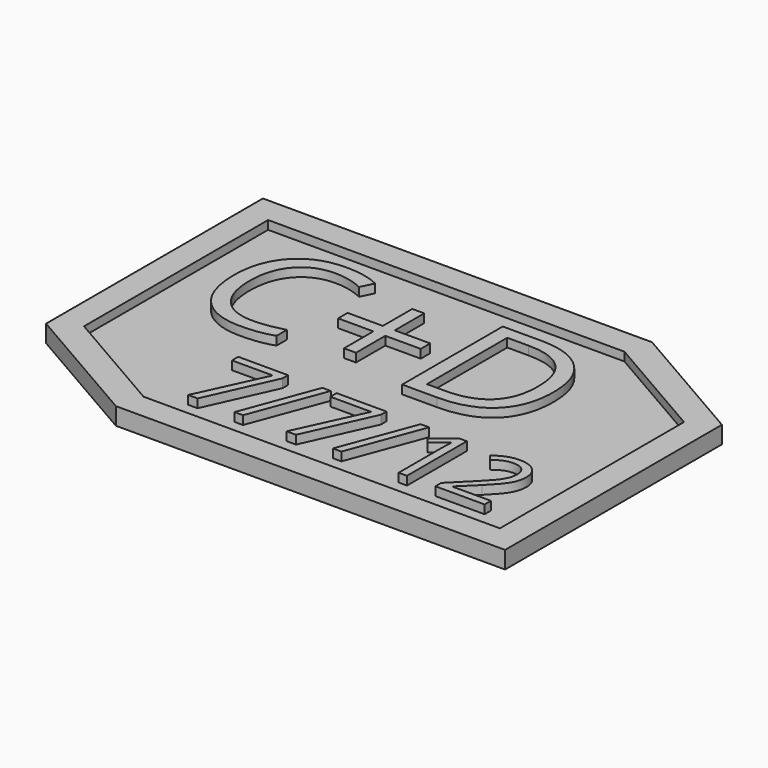
from build123d import *

# Parameters (mm, degrees)
F0_W           = 60
F0_H           = 40
F1_DEPTH       = 1
F2_SIZE2       = 8.6602540378
F2_SIZE        = 15
F2_2_SIZE2     = 8.6602540378
F2_2_SIZE      = 15
F4_DEPTH       = 1
F5_TEXT_SIZE   = 20.360840588
F5_TEXT_SIZE_2 = 12.11661535
F6_DEPTH       = 1


# Not quite as in the source:
# - Text() gives the source's letters only with a copy of the font that has no kerning and outlines rounded to 1/6400 em; it was checked with that copy


with BuildPart() as f1:
    # F0 (on Top) → F1 (new body)
    with BuildSketch(Plane.XY):
        with Locations((30, 20)):
            Rectangle(F0_W, F0_H)
    extrude(amount=F1_DEPTH)

    # F2
    f2_edges = [f1.edges().sort_by_distance(p)[0] for p in [
        (0, 0, 0.5),
    ]]
    f2_side = f1.faces().sort_by_distance((30, 0, 0.5))[0]
    chamfer(f2_edges, length=F2_SIZE, length2=F2_SIZE2, reference=f2_side)

    # F2#2
    f2_2_edges = [f1.edges().sort_by_distance(p)[0] for p in [
        (60, 40, 0.5),
    ]]
    f2_2_side = f1.faces().sort_by_distance((30, 40, 0.5))[0]
    chamfer(f2_2_edges, length=F2_2_SIZE, length2=F2_2_SIZE2, reference=f2_2_side)

    # F3 (on face) → F4 (join)
    with BuildSketch(Plane.XY.offset(1)):
        Polygon((15, 0), (60, 0), (60, 31.3397459622), (45, 40), (0, 40), (0, 8.6602540378), align=None)
        Polygon((57, 3), (15.8038475773, 3), (3, 10.3923048454), (3, 37), (44.1961524227, 37), (57, 29.6076951546), align=None, mode=Mode.SUBTRACT)
    extrude(amount=F4_DEPTH)

    # F5 (on face) → F6 (join)
    with BuildSketch(Plane.XY.offset(1)):
        with Locations((6.0659060255, 19.4407235831)):
            Text('C+D', F5_TEXT_SIZE, font='Open Sans', text_align=(TextAlign.LEFT, TextAlign.BOTTOM))
        with Locations((17.0456878841, 5.783108063)):
            Text('7/7/12', F5_TEXT_SIZE_2, font='Open Sans', text_align=(TextAlign.LEFT, TextAlign.BOTTOM))
    extrude(amount=F6_DEPTH)


solid = f1.part
